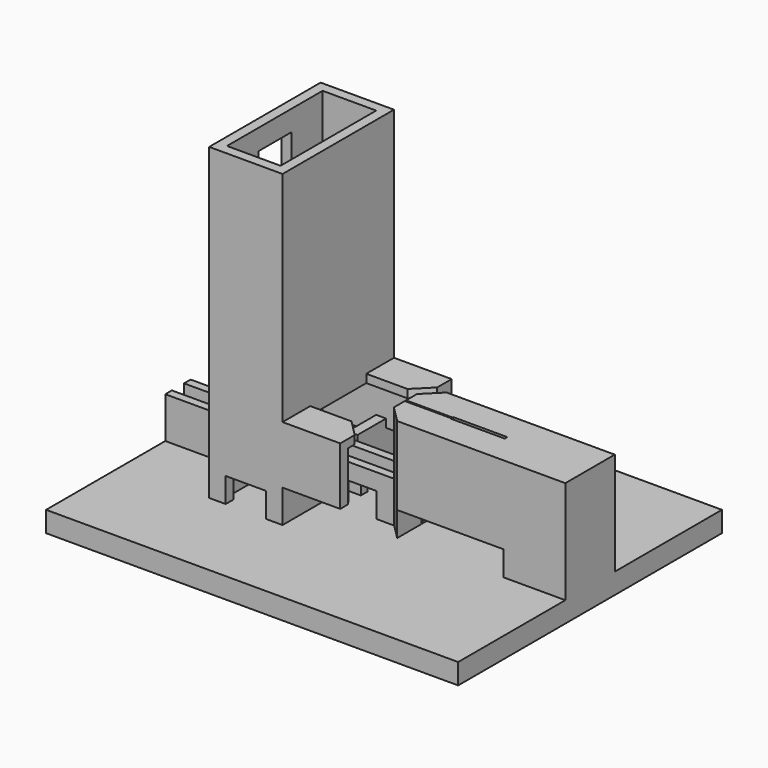
from build123d import *

# Parameters (mm, degrees)
F0_W          = 11.303
F0_H          = 21.463
F0_W_2        = 8.255
F0_H_2        = 18.415
F1_DEPTH      = 50.8
F2_W          = 18.415
F2_H          = 6.35
F3_DEPTH      = 12.7
F4_W          = 6.35
F4_H          = 31.75
F5_DEPTH      = 25.4
F6_W          = 63.5
F6_H          = 50.8
F7_DEPTH      = 3.175
F8_W          = 28.448
F8_H          = 9.525
F9_DEPTH      = 15.875
F11_DEPTH     = 15.875
F12_W         = 35.052
F12_H         = 1.27
F13_DEPTH     = 6.35
F14_W         = 1.27
F14_H         = 1.27
F14_W_2       = 2.3495
F15_DEPTH     = 24.7025
F16_W         = 6.223
F16_H         = 3.81
F16_W_2       = 5.2705
F16_W_3       = 16.383
F17_DEPTH     = 36.1325
F19_DEPTH     = 8.89
F20_T1_DEPTH  = 14.3341495789
F20_T6_DEPTH  = 22.4070747894
F20_T11_DEPTH = 28.9391495789
F20_T16_DEPTH = 22.4070747894
F20_T21_DEPTH = 28.9391495789


# Not quite as in the source:
# - a fillet or chamfer that OpenCascade refuses, or shapes differently, is made with other operations: its cross-section is extruded or revolved along the edge and cut away or added


with BuildPart() as f1:
    # F0 (on Top) → F1 (new body)
    with BuildSketch(Plane.XY):
        Rectangle(F0_W, F0_H)
        Rectangle(F0_W_2, F0_H_2, mode=Mode.SUBTRACT)
    extrude(amount=F1_DEPTH)

    # F2 (on Right) → F3 (cut, symmetric)
    with BuildSketch(Plane.YZ):
        with Locations((0, 12.7)):
            Rectangle(F2_W, F2_H)
    extrude(amount=F3_DEPTH, both=True, mode=Mode.SUBTRACT)

    # F4 (on Right) → F5 (cut)
    with BuildSketch(Plane.YZ):
        with Locations((0, 31.75)):
            Rectangle(F4_W, F4_H)
    extrude(amount=-F5_DEPTH, mode=Mode.SUBTRACT)

    # F6 (on Top) → F7 (join)
    with BuildSketch(Plane.XY):
        with Locations((12.7, 0)):
            Rectangle(F6_W, F6_H)
    extrude(amount=F7_DEPTH)

    # F8 (on face) → F9 (join)
    with BuildSketch(Plane.XY.offset(3.175)):
        with Locations((30.226, 0)):
            Rectangle(F8_W, F8_H)
    extrude(amount=F9_DEPTH)

    # F10 (on face) → F11 (cut, through all)
    with BuildSketch(Plane.XY.offset(19.05)):
        Polygon((11.684, 0.127), (11.684, -0.127), (23.1648, -0.127), (23.1648, -0.254), (31.496, -0.254), (31.496, 0.254), (23.1648, 0.254), (23.1648, 0.127), align=None)
    extrude(amount=-F11_DEPTH, mode=Mode.SUBTRACT)

    # F12 (on face) → F13 (join)
    with BuildSketch(Plane.XY.offset(3.175)):
        with Locations((-1.524, 1.80975)):
            Rectangle(F12_W, F12_H)
        with Locations((-1.524, -1.80975)):
            Rectangle(F12_W, F12_H)
    extrude(amount=F13_DEPTH)

    # F14 (on face) → F15 (cut, through all)
    with BuildSketch(Plane.YZ.offset(5.6515)):
        with Locations((-3.07975, 8.89)):
            Rectangle(F14_W, F14_H)
        with Locations((0, 8.89)):
            Rectangle(F14_W_2, F14_H)
        with Locations((3.07975, 8.89)):
            Rectangle(F14_W, F14_H)
    extrude(amount=-F15_DEPTH, mode=Mode.SUBTRACT)

    # F16 (on face) → F17 (cut, through all)
    with BuildSketch(Plane.XZ.offset(10.7315)):
        with Locations((0, 5.08)):
            Rectangle(F16_W, F16_H)
        with Locations((10.82675, 5.08)):
            Rectangle(F16_W_2, F16_H)
        with Locations((26.7335, 5.08)):
            Rectangle(F16_W_3, F16_H)
    extrude(amount=-F17_DEPTH, mode=Mode.SUBTRACT)

    # F18 (on face) → F19 (join)
    with BuildSketch(Plane.YZ.offset(5.6515)):
        Polygon((-9.2075, 15.875), (-5.3975, 15.875), (-5.3975, 17.145), (-10.7315, 17.145), (-10.7315, 8.255), (-9.2075, 8.255), align=None)
        Polygon((10.7315, 17.145), (5.3975, 17.145), (5.3975, 15.875), (9.2075, 15.875), (9.2075, 8.255), (10.7315, 8.255), align=None)
    extrude(amount=F19_DEPTH)

    # F20: chamfer of 2.54 on 4 edges, made by hand

    # F20_s2 → F20_t1 (cut)
    with BuildSketch(Plane.XY.offset(9.3429252106)):
        Polygon((14.5415, 7.9375), (12.0015, 5.3975), (14.5415, 5.3975), align=None)
        Polygon((12.0015, -5.3975), (14.5415, -7.9375), (14.5415, -5.3975), align=None)
    extrude(amount=F20_T1_DEPTH, mode=Mode.SUBTRACT)


with BuildPart() as f20_tool4:
    # F20_s5 → F20_t6 (new body)
    with BuildSketch(Plane.XY.offset(3.175)):
        Polygon((16.002, -2.2225), (18.542, -4.7625), (16.002, -4.7625), align=None)
    extrude(amount=F20_T6_DEPTH)

    split(bisect_by=Plane.XZ.offset(2.44475), keep=Keep.TOP)


with BuildPart() as f1_1:
    add(f1.part)

    # F20_t3: cut F20_tool4
    add(f20_tool4.part, mode=Mode.SUBTRACT)


with BuildPart() as f20_tool9:
    # F20_s10 → F20_t11 (new body)
    with BuildSketch(Plane.XY.offset(-3.3570747894)):
        Polygon((16.002, -2.2225), (18.542, -4.7625), (16.002, -4.7625), align=None)
    extrude(amount=F20_T11_DEPTH)

    split(bisect_by=Plane.XY.offset(9.525), keep=Keep.TOP)


with BuildPart() as f1_2:
    add(f1_1.part)

    # F20_t8: cut F20_tool9
    add(f20_tool9.part, mode=Mode.SUBTRACT)


with BuildPart() as f20_tool14:
    # F20_s15 → F20_t16 (new body)
    with BuildSketch(Plane.XY.offset(3.175)):
        Polygon((16.002, 2.2225), (18.542, 4.7625), (16.002, 4.7625), align=None)
    extrude(amount=F20_T16_DEPTH)

    split(bisect_by=Plane.XZ.offset(-2.44475), keep=Keep.BOTTOM)


with BuildPart() as f1_3:
    add(f1_2.part)

    # F20_t13: cut F20_tool14
    add(f20_tool14.part, mode=Mode.SUBTRACT)


with BuildPart() as f20_tool19:
    # F20_s20 → F20_t21 (new body)
    with BuildSketch(Plane.XY.offset(-3.3570747894)):
        Polygon((16.002, 2.2225), (18.542, 4.7625), (16.002, 4.7625), align=None)
    extrude(amount=F20_T21_DEPTH)

    split(bisect_by=Plane.XY.offset(9.525), keep=Keep.TOP)


with BuildPart() as f1_4:
    add(f1_3.part)

    # F20_t18: cut F20_tool19
    add(f20_tool19.part, mode=Mode.SUBTRACT)


solid = f1_4.part
